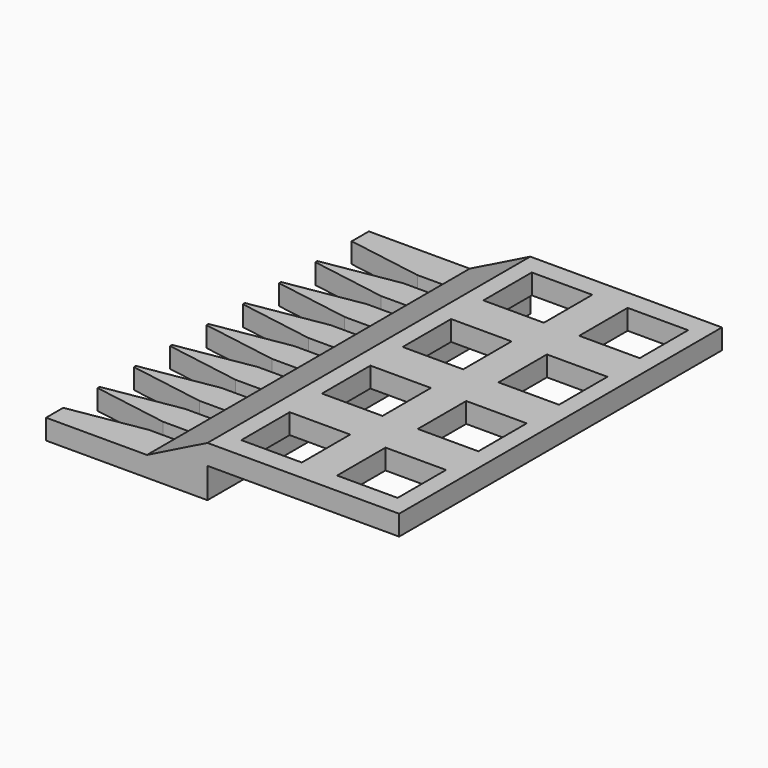
from build123d import *

# Parameters (mm, degrees)
F1_DEPTH   = 80
F2_W       = 20
F2_H       = 3.5
F3_DEPTH   = 4.001
F4_SIZE2   = 11.99999
F4_SIZE    = 5.99999
F5_SIZE2   = 2.5
F5_SIZE    = 15
F5_2_SIZE2 = 2.5
F5_2_SIZE  = 15
F5_3_SIZE2 = 2.5
F5_3_SIZE  = 15
F5_4_SIZE2 = 2.5
F5_4_SIZE  = 15
F5_5_SIZE2 = 2.5
F5_5_SIZE  = 15
F5_6_SIZE2 = 2.5
F5_6_SIZE  = 15
F5_7_SIZE2 = 2.5
F5_7_SIZE  = 15
F5_8_SIZE2 = 2.5
F5_8_SIZE  = 15
F6_SIZE2   = 2.5
F6_SIZE    = 15
F6_2_SIZE2 = 2.5
F6_2_SIZE  = 15
F6_3_SIZE2 = 2.5
F6_3_SIZE  = 15
F6_4_SIZE2 = 2.5
F6_4_SIZE  = 15
F6_5_SIZE2 = 2.5
F6_5_SIZE  = 15
F6_6_SIZE2 = 2.5
F6_6_SIZE  = 15
F6_7_SIZE2 = 2.5
F6_7_SIZE  = 15
F6_8_SIZE2 = 2.5
F6_8_SIZE  = 15
F7_W       = 30
F7_H       = 80
F8_DEPTH   = 25
F9_W       = 12
F9_H       = 12
F10_DEPTH  = 10.001


# Not quite as in the source:
# - a fillet or chamfer is up to 0.001 mm smaller than in the source, because OpenCascade refuses the exact size


with BuildPart() as f1:
    # F0 (on Front) → F1 (new body)
    with BuildSketch(Plane.XZ):
        Polygon((0, 4), (0, 0), (32, 0), (32, 6), (100, 6), (100, 10), (20, 10), (20, 4), align=None)
    extrude(amount=F1_DEPTH)

    # F2 (on face) → F3 (cut, through all)
    with BuildSketch(Plane.XY.offset(4)):
        with Locations((10, -35.5)):
            Rectangle(F2_W, F2_H)
        with Locations((10, -26.5)):
            Rectangle(F2_W, F2_H)
        with Locations((10, -17.5)):
            Rectangle(F2_W, F2_H)
        with Locations((10, -8.5)):
            Rectangle(F2_W, F2_H)
        with Locations((10, -71.5)):
            Rectangle(F2_W, F2_H)
        with Locations((10, -53.5)):
            Rectangle(F2_W, F2_H)
        with Locations((10, -44.5)):
            Rectangle(F2_W, F2_H)
        with Locations((10, -62.5)):
            Rectangle(F2_W, F2_H)
    extrude(amount=-F3_DEPTH, mode=Mode.SUBTRACT)

    # F4 (size 6 and 12 in the source; OpenCascade refuses exactly that, so slightly less here)
    f4_edges = [f1.edges().sort_by_distance(p)[0] for p in [
        (20, -40, 10),
    ]]
    f4_side = f1.faces().sort_by_distance((20, -40, 6.054054))[0]
    chamfer(f4_edges, length=F4_SIZE, length2=F4_SIZE2, reference=f4_side)

    # F5
    f5_edges = [f1.edges().sort_by_distance(p)[0] for p in [
        (0, -6.75, 2),
    ]]
    f5_side = f1.faces().sort_by_distance((10, -6.75, 2))[0]
    chamfer(f5_edges, length=F5_SIZE, length2=F5_SIZE2, reference=f5_side)

    # F5#2
    f5_2_edges = [f1.edges().sort_by_distance(p)[0] for p in [
        (0, -69.75, 2),
    ]]
    f5_2_side = f1.faces().sort_by_distance((10, -69.75, 2))[0]
    chamfer(f5_2_edges, length=F5_2_SIZE, length2=F5_2_SIZE2, reference=f5_2_side)

    # F5#3
    f5_3_edges = [f1.edges().sort_by_distance(p)[0] for p in [
        (0, -15.75, 2),
    ]]
    f5_3_side = f1.faces().sort_by_distance((10, -15.75, 2))[0]
    chamfer(f5_3_edges, length=F5_3_SIZE, length2=F5_3_SIZE2, reference=f5_3_side)

    # F5#4
    f5_4_edges = [f1.edges().sort_by_distance(p)[0] for p in [
        (0, -60.75, 2),
    ]]
    f5_4_side = f1.faces().sort_by_distance((10, -60.75, 2))[0]
    chamfer(f5_4_edges, length=F5_4_SIZE, length2=F5_4_SIZE2, reference=f5_4_side)

    # F5#5
    f5_5_edges = [f1.edges().sort_by_distance(p)[0] for p in [
        (0, -24.75, 2),
    ]]
    f5_5_side = f1.faces().sort_by_distance((10, -24.75, 2))[0]
    chamfer(f5_5_edges, length=F5_5_SIZE, length2=F5_5_SIZE2, reference=f5_5_side)

    # F5#6
    f5_6_edges = [f1.edges().sort_by_distance(p)[0] for p in [
        (0, -51.75, 2),
    ]]
    f5_6_side = f1.faces().sort_by_distance((10, -51.75, 2))[0]
    chamfer(f5_6_edges, length=F5_6_SIZE, length2=F5_6_SIZE2, reference=f5_6_side)

    # F5#7
    f5_7_edges = [f1.edges().sort_by_distance(p)[0] for p in [
        (0, -33.75, 2),
    ]]
    f5_7_side = f1.faces().sort_by_distance((10, -33.75, 2))[0]
    chamfer(f5_7_edges, length=F5_7_SIZE, length2=F5_7_SIZE2, reference=f5_7_side)

    # F5#8
    f5_8_edges = [f1.edges().sort_by_distance(p)[0] for p in [
        (0, -42.75, 2),
    ]]
    f5_8_side = f1.faces().sort_by_distance((10, -42.75, 2))[0]
    chamfer(f5_8_edges, length=F5_8_SIZE, length2=F5_8_SIZE2, reference=f5_8_side)

    # F6
    f6_edges = [f1.edges().sort_by_distance(p)[0] for p in [
        (0, -37.25, 2),
    ]]
    f6_side = f1.faces().sort_by_distance((10, -37.25, 2))[0]
    chamfer(f6_edges, length=F6_SIZE, length2=F6_SIZE2, reference=f6_side)

    # F6#2
    f6_2_edges = [f1.edges().sort_by_distance(p)[0] for p in [
        (0, -46.25, 2),
    ]]
    f6_2_side = f1.faces().sort_by_distance((10, -46.25, 2))[0]
    chamfer(f6_2_edges, length=F6_2_SIZE, length2=F6_2_SIZE2, reference=f6_2_side)

    # F6#3
    f6_3_edges = [f1.edges().sort_by_distance(p)[0] for p in [
        (0, -28.25, 2),
    ]]
    f6_3_side = f1.faces().sort_by_distance((10, -28.25, 2))[0]
    chamfer(f6_3_edges, length=F6_3_SIZE, length2=F6_3_SIZE2, reference=f6_3_side)

    # F6#4
    f6_4_edges = [f1.edges().sort_by_distance(p)[0] for p in [
        (0, -55.25, 2),
    ]]
    f6_4_side = f1.faces().sort_by_distance((10, -55.25, 2))[0]
    chamfer(f6_4_edges, length=F6_4_SIZE, length2=F6_4_SIZE2, reference=f6_4_side)

    # F6#5
    f6_5_edges = [f1.edges().sort_by_distance(p)[0] for p in [
        (0, -19.25, 2),
    ]]
    f6_5_side = f1.faces().sort_by_distance((10, -19.25, 2))[0]
    chamfer(f6_5_edges, length=F6_5_SIZE, length2=F6_5_SIZE2, reference=f6_5_side)

    # F6#6
    f6_6_edges = [f1.edges().sort_by_distance(p)[0] for p in [
        (0, -64.25, 2),
    ]]
    f6_6_side = f1.faces().sort_by_distance((10, -64.25, 2))[0]
    chamfer(f6_6_edges, length=F6_6_SIZE, length2=F6_6_SIZE2, reference=f6_6_side)

    # F6#7
    f6_7_edges = [f1.edges().sort_by_distance(p)[0] for p in [
        (0, -10.25, 2),
    ]]
    f6_7_side = f1.faces().sort_by_distance((10, -10.25, 2))[0]
    chamfer(f6_7_edges, length=F6_7_SIZE, length2=F6_7_SIZE2, reference=f6_7_side)

    # F6#8
    f6_8_edges = [f1.edges().sort_by_distance(p)[0] for p in [
        (0, -73.25, 2),
    ]]
    f6_8_side = f1.faces().sort_by_distance((10, -73.25, 2))[0]
    chamfer(f6_8_edges, length=F6_8_SIZE, length2=F6_8_SIZE2, reference=f6_8_side)

    # F7 (on face) → F8 (cut)
    with BuildSketch(Plane.XY.offset(10)):
        with Locations((85, -40)):
            Rectangle(F7_W, F7_H)
    extrude(amount=-F8_DEPTH, mode=Mode.SUBTRACT)

    # F9 (on face) → F10 (cut, through all)
    with BuildSketch(Plane.XY.offset(10)):
        with Locations((41.5, -10)):
            Rectangle(F9_W, F9_H)
        with Locations((41.5, -30)):
            Rectangle(F9_W, F9_H)
        with Locations((41.5, -50)):
            Rectangle(F9_W, F9_H)
        with Locations((41.5, -70)):
            Rectangle(F9_W, F9_H)
        with Locations((60.5, -30)):
            Rectangle(F9_W, F9_H)
        with Locations((60.5, -70)):
            Rectangle(F9_W, F9_H)
        with Locations((60.5, -10)):
            Rectangle(F9_W, F9_H)
        with Locations((60.5, -50)):
            Rectangle(F9_W, F9_H)
    extrude(amount=-F10_DEPTH, mode=Mode.SUBTRACT)


solid = f1.part
